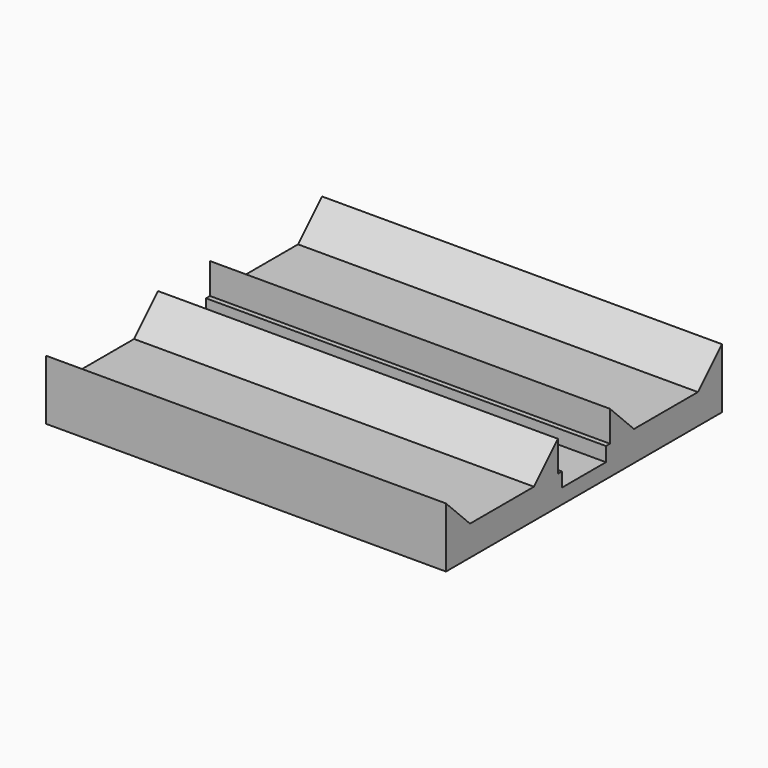
from build123d import *

# Parameters (mm, degrees)
F0_W     = 20
F0_H     = 34.5
F1_DEPTH = 6
F2_DEPTH = 20
F3_W     = 5.5
F3_H     = 3.0757111441
F3_W_2   = 0.5
F3_H_2   = 1.4242888559
F4_DEPTH = 50
F5_W     = 8
F5_H     = 3
F6_DEPTH = 50
F7_SIZE  = 2.99999


# Not quite as in the source:
# - a fillet or chamfer is up to 0.001 mm smaller than in the source, because OpenCascade refuses the exact size


with BuildPart() as f1:
    # F0 (on Top) → F1 (new body)
    with BuildSketch(Plane.XY):
        with Locations((10, 17.25)):
            Rectangle(F0_W, F0_H)
    extrude(amount=F1_DEPTH)

    # F2 (add): a face of the model
    f2_faces = [f1.faces().sort_by_distance(p)[0] for p in [
        (20, 17.25, 3),
    ]]
    extrude(f2_faces, amount=F2_DEPTH)

    # F3 (on face) → F4 (cut)
    with BuildSketch(Plane(origin=(0, 0, 0), x_dir=(0, -1, 0), z_dir=(-1, 0, 0))):
        Polygon((-20, 6.5), (-14.5, 6.5), (-14.5, 6), (-14, 6), (-14, 9.0350331739), (-20.5, 9.0350331739), (-20.5, 6), (-20, 6), align=None)
        with Locations((-17.25, 4.4621444279)):
            Rectangle(F3_W, F3_H)
        with Locations((-14.25, 4.4621444279)):
            Rectangle(F3_W_2, F3_H)
        with Locations((-20.25, 4.4621444279)):
            Rectangle(F3_W_2, F3_H)
        with Locations((-17.25, 2.2121444279)):
            Rectangle(F3_W, F3_H_2)
    extrude(amount=-F4_DEPTH, mode=Mode.SUBTRACT)

    # F5 (on face) → F6 (cut)
    with BuildSketch(Plane(origin=(0, 0, 0), x_dir=(0, -1, 0), z_dir=(-1, 0, 0))):
        with Locations((-27.5, 4.5)):
            Rectangle(F5_W, F5_H)
        with Locations((-7, 4.5)):
            Rectangle(F5_W, F5_H)
    extrude(amount=-F6_DEPTH, mode=Mode.SUBTRACT)

    # F7 (size 3 in the source; OpenCascade refuses exactly that, so slightly less here)
    f7_edges = [f1.edges().sort_by_distance(p)[0] for p in [
        (20, 11, 6),
        (20, 3, 6),
        (20, 31.5, 6),
        (20, 23.5, 6),
    ]]
    chamfer(f7_edges, length=F7_SIZE)


solid = f1.part
